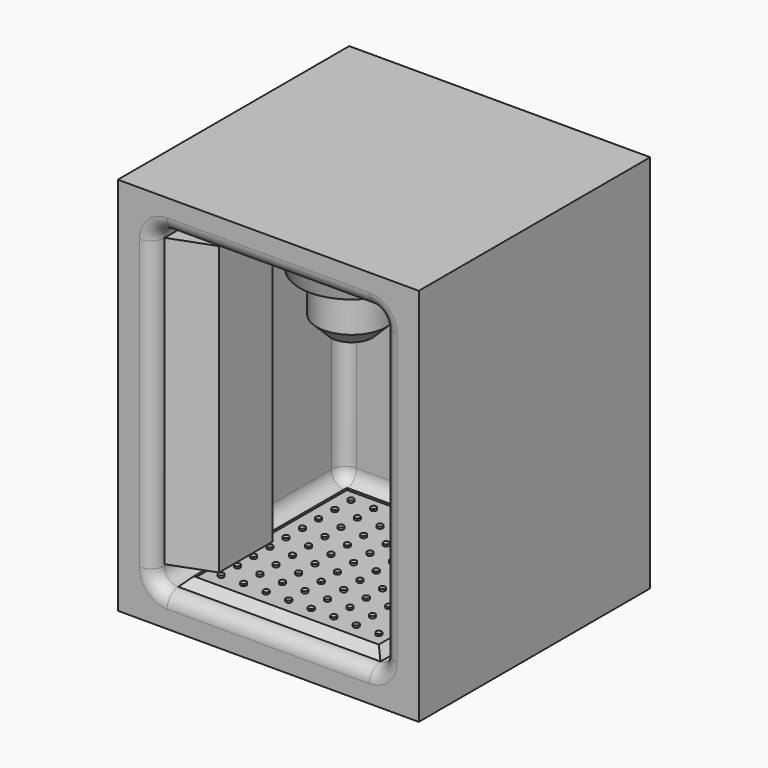
from build123d import *

# Parameters (mm, degrees)
F0_W      = 108.2055345178
F0_H      = 136.4547163248
F1_DEPTH  = 52
F2_W      = 82.6906114817
F2_H      = 113.8212010264
F3_DEPTH  = 85
F4_R      = 5
F8_W      = 15.0986835361
F8_H      = 103.3223718405
F9_DEPTH  = 29.6
F11_DEPTH = 104.4
F12_DEPTH = 12.7
F13_SIZE  = 5
F3_FACE_W = 72.6906114817
F3_FACE_H = 75
F14_DEPTH = 3.1
F14_TAPER = 45
F15_W     = 66.4906114817
F15_H     = 68.8
F15_R     = 1
F16_DEPTH = 0.7


with BuildPart() as f1:
    # F0 (on Front) → F1 (new body, symmetric)
    with BuildSketch(Plane.XZ):
        Rectangle(F0_W, F0_H)
    extrude(amount=F1_DEPTH, both=True)

    # F2 (on face) → F3 (cut)
    with BuildSketch(Plane.XZ.offset(52)):
        Rectangle(F2_W, F2_H)
    extrude(amount=-F3_DEPTH, mode=Mode.SUBTRACT)

    # F4
    f4_edges = [f1.edges().sort_by_distance(p)[0] for p in [
        (41.345306, -9.5, 56.910601),
        (-41.345306, -9.5, 56.910601),
        (0, -52, 56.910601),
        (0, 33, 56.910601),
        (-41.345306, -9.5, -56.910601),
        (41.345306, -9.5, -56.910601),
        (0, -52, -56.910601),
        (0, 33, -56.910601),
        (41.345306, -52, 0),
        (41.345306, 33, 0),
        (-41.345306, 33, 0),
        (-41.345306, -52, 0),
    ]]
    fillet(f4_edges, radius=F4_R)


with BuildPart() as f6:
    # F5 (on Right) → F6 (revolve)
    with BuildSketch(Plane.YZ):
        Polygon((8.3307297271, 56.9845885038), (-14.5597765222, 56.9845885038), (-14.5597765222, 35.6844794005), (-2.0613675006, 35.6844794005), (-2.0613675006, 42.3737689853), (4.1059157182, 42.3737689853), align=None)
    revolve(axis=Axis((0, -14.5597765222, 46.3345339522), (0, 0, -1)))

    # F12 (add): a face of the model
    f12_faces = [f6.faces().sort_by_distance(p)[0] for p in [
        (0, -14.5597765222, 35.6844794005),
    ]]
    extrude(f12_faces, amount=F12_DEPTH)

    # F13
    f13_edges = [f6.edges().sort_by_distance(p)[0] for p in [
        (0, -27.058186, 22.984479),
    ]]
    chamfer(f13_edges, length=F13_SIZE)


with BuildPart() as f9:
    # F8 (on offset) → F9 (new body)
    with BuildSketch(Plane.XZ.offset(47)):
        with Locations((-33.7500013411, 0.2960525453)):
            Rectangle(F8_W, F8_H)
    extrude(amount=-F9_DEPTH)

    # F10 (on face) → F11 (cut)
    with BuildSketch(Plane.XY.offset(51.9572384655)):
        Polygon((-26.2006595731, -41.4010522253), (-41.2993431091, -47), (-26.2006595731, -47), align=None)
    extrude(amount=-F11_DEPTH, mode=Mode.SUBTRACT)


with BuildPart() as f14:
    # F3_face (on face) → F14 (new body)
    with BuildSketch(Plane(origin=(0, -9.5, -56.9106005132), x_dir=(1, 0, 0), z_dir=(0, 0, 1))):
        Rectangle(F3_FACE_W, F3_FACE_H)
    extrude(amount=F14_DEPTH, taper=F14_TAPER)

    # F15 (on face) → F16 (cut)
    with BuildSketch(Plane.XY.offset(-53.8106005132)):
        with Locations((0, -9.5)):
            Rectangle(F15_W, F15_H)
        with Locations((-28.0926923715, -38.0783945817)):
            Circle(F15_R, mode=Mode.SUBTRACT)
        with Locations((-19.9926923715, -38.0783945817)):
            Circle(F15_R, mode=Mode.SUBTRACT)
        with Locations((-28.0943763485, -30.7783947759)):
            Circle(F15_R, mode=Mode.SUBTRACT)
        with Locations((-19.9943763485, -30.7783947759)):
            Circle(F15_R, mode=Mode.SUBTRACT)
        with Locations((-11.8926923715, -38.0783945817)):
            Circle(F15_R, mode=Mode.SUBTRACT)
        with Locations((-3.7926923715, -38.0783945817)):
            Circle(F15_R, mode=Mode.SUBTRACT)
        with Locations((-11.8943763485, -30.7783947759)):
            Circle(F15_R, mode=Mode.SUBTRACT)
        with Locations((-3.7943763485, -30.7783947759)):
            Circle(F15_R, mode=Mode.SUBTRACT)
        with Locations((-28.0960603254, -23.4783949702)):
            Circle(F15_R, mode=Mode.SUBTRACT)
        with Locations((-19.9960603254, -23.4783949702)):
            Circle(F15_R, mode=Mode.SUBTRACT)
        with Locations((-28.0977443024, -16.1783951644)):
            Circle(F15_R, mode=Mode.SUBTRACT)
        with Locations((-19.9977443024, -16.1783951644)):
            Circle(F15_R, mode=Mode.SUBTRACT)
        with Locations((-11.8960603254, -23.4783949702)):
            Circle(F15_R, mode=Mode.SUBTRACT)
        with Locations((-3.7960603254, -23.4783949702)):
            Circle(F15_R, mode=Mode.SUBTRACT)
        with Locations((-11.8977443024, -16.1783951644)):
            Circle(F15_R, mode=Mode.SUBTRACT)
        with Locations((-3.7977443024, -16.1783951644)):
            Circle(F15_R, mode=Mode.SUBTRACT)
        with Locations((4.3073076285, -38.0783945817)):
            Circle(F15_R, mode=Mode.SUBTRACT)
        with Locations((12.4073076285, -38.0783945817)):
            Circle(F15_R, mode=Mode.SUBTRACT)
        with Locations((4.3056236515, -30.7783947759)):
            Circle(F15_R, mode=Mode.SUBTRACT)
        with Locations((12.4056236515, -30.7783947759)):
            Circle(F15_R, mode=Mode.SUBTRACT)
        with Locations((20.5073076285, -38.0783945817)):
            Circle(F15_R, mode=Mode.SUBTRACT)
        with Locations((28.6073076285, -38.0783945817)):
            Circle(F15_R, mode=Mode.SUBTRACT)
        with Locations((20.5056236515, -30.7783947759)):
            Circle(F15_R, mode=Mode.SUBTRACT)
        with Locations((28.6056236515, -30.7783947759)):
            Circle(F15_R, mode=Mode.SUBTRACT)
        with Locations((4.3039396746, -23.4783949702)):
            Circle(F15_R, mode=Mode.SUBTRACT)
        with Locations((12.4039396746, -23.4783949702)):
            Circle(F15_R, mode=Mode.SUBTRACT)
        with Locations((4.3022556976, -16.1783951644)):
            Circle(F15_R, mode=Mode.SUBTRACT)
        with Locations((12.4022556976, -16.1783951644)):
            Circle(F15_R, mode=Mode.SUBTRACT)
        with Locations((20.5039396746, -23.4783949702)):
            Circle(F15_R, mode=Mode.SUBTRACT)
        with Locations((28.6039396746, -23.4783949702)):
            Circle(F15_R, mode=Mode.SUBTRACT)
        with Locations((20.5022556976, -16.1783951644)):
            Circle(F15_R, mode=Mode.SUBTRACT)
        with Locations((28.6022556976, -16.1783951644)):
            Circle(F15_R, mode=Mode.SUBTRACT)
        with Locations((-28.0994282793, -8.8783953586)):
            Circle(F15_R, mode=Mode.SUBTRACT)
        with Locations((-28.1011122563, -1.5783955529)):
            Circle(F15_R, mode=Mode.SUBTRACT)
        with Locations((-19.9994282793, -8.8783953586)):
            Circle(F15_R, mode=Mode.SUBTRACT)
        with Locations((-20.0011122563, -1.5783955529)):
            Circle(F15_R, mode=Mode.SUBTRACT)
        with Locations((-28.1027962333, 5.7216042529)):
            Circle(F15_R, mode=Mode.SUBTRACT)
        with Locations((-20.0027962333, 5.7216042529)):
            Circle(F15_R, mode=Mode.SUBTRACT)
        with Locations((-11.8994282793, -8.8783953586)):
            Circle(F15_R, mode=Mode.SUBTRACT)
        with Locations((-11.9011122563, -1.5783955529)):
            Circle(F15_R, mode=Mode.SUBTRACT)
        with Locations((-3.7994282793, -8.8783953586)):
            Circle(F15_R, mode=Mode.SUBTRACT)
        with Locations((-3.8011122563, -1.5783955529)):
            Circle(F15_R, mode=Mode.SUBTRACT)
        with Locations((-11.9027962333, 5.7216042529)):
            Circle(F15_R, mode=Mode.SUBTRACT)
        with Locations((-3.8027962333, 5.7216042529)):
            Circle(F15_R, mode=Mode.SUBTRACT)
        with Locations((-28.1044802102, 13.0216040587)):
            Circle(F15_R, mode=Mode.SUBTRACT)
        with Locations((-20.0044802102, 13.0216040587)):
            Circle(F15_R, mode=Mode.SUBTRACT)
        with Locations((-28.1061641872, 20.3216038644)):
            Circle(F15_R, mode=Mode.SUBTRACT)
        with Locations((-20.0061641872, 20.3216038644)):
            Circle(F15_R, mode=Mode.SUBTRACT)
        with Locations((-11.9044802102, 13.0216040587)):
            Circle(F15_R, mode=Mode.SUBTRACT)
        with Locations((-3.8044802102, 13.0216040587)):
            Circle(F15_R, mode=Mode.SUBTRACT)
        with Locations((-11.9061641872, 20.3216038644)):
            Circle(F15_R, mode=Mode.SUBTRACT)
        with Locations((-3.8061641872, 20.3216038644)):
            Circle(F15_R, mode=Mode.SUBTRACT)
        with Locations((4.3005717207, -8.8783953586)):
            Circle(F15_R, mode=Mode.SUBTRACT)
        with Locations((4.2988877437, -1.5783955529)):
            Circle(F15_R, mode=Mode.SUBTRACT)
        with Locations((12.4005717207, -8.8783953586)):
            Circle(F15_R, mode=Mode.SUBTRACT)
        with Locations((12.3988877437, -1.5783955529)):
            Circle(F15_R, mode=Mode.SUBTRACT)
        with Locations((4.2972037667, 5.7216042529)):
            Circle(F15_R, mode=Mode.SUBTRACT)
        with Locations((12.3972037667, 5.7216042529)):
            Circle(F15_R, mode=Mode.SUBTRACT)
        with Locations((20.5005717207, -8.8783953586)):
            Circle(F15_R, mode=Mode.SUBTRACT)
        with Locations((20.4988877437, -1.5783955529)):
            Circle(F15_R, mode=Mode.SUBTRACT)
        with Locations((28.6005717207, -8.8783953586)):
            Circle(F15_R, mode=Mode.SUBTRACT)
        with Locations((28.5988877437, -1.5783955529)):
            Circle(F15_R, mode=Mode.SUBTRACT)
        with Locations((20.4972037667, 5.7216042529)):
            Circle(F15_R, mode=Mode.SUBTRACT)
        with Locations((28.5972037667, 5.7216042529)):
            Circle(F15_R, mode=Mode.SUBTRACT)
        with Locations((4.2955197898, 13.0216040587)):
            Circle(F15_R, mode=Mode.SUBTRACT)
        with Locations((12.3955197898, 13.0216040587)):
            Circle(F15_R, mode=Mode.SUBTRACT)
        with Locations((4.2938358128, 20.3216038644)):
            Circle(F15_R, mode=Mode.SUBTRACT)
        with Locations((12.3938358128, 20.3216038644)):
            Circle(F15_R, mode=Mode.SUBTRACT)
        with Locations((20.4955197898, 13.0216040587)):
            Circle(F15_R, mode=Mode.SUBTRACT)
        with Locations((28.5955197898, 13.0216040587)):
            Circle(F15_R, mode=Mode.SUBTRACT)
        with Locations((20.4938358128, 20.3216038644)):
            Circle(F15_R, mode=Mode.SUBTRACT)
        with Locations((28.5938358128, 20.3216038644)):
            Circle(F15_R, mode=Mode.SUBTRACT)
    extrude(amount=-F16_DEPTH, mode=Mode.SUBTRACT)


solid = Compound([f1.part, f6.part, f9.part, f14.part])
